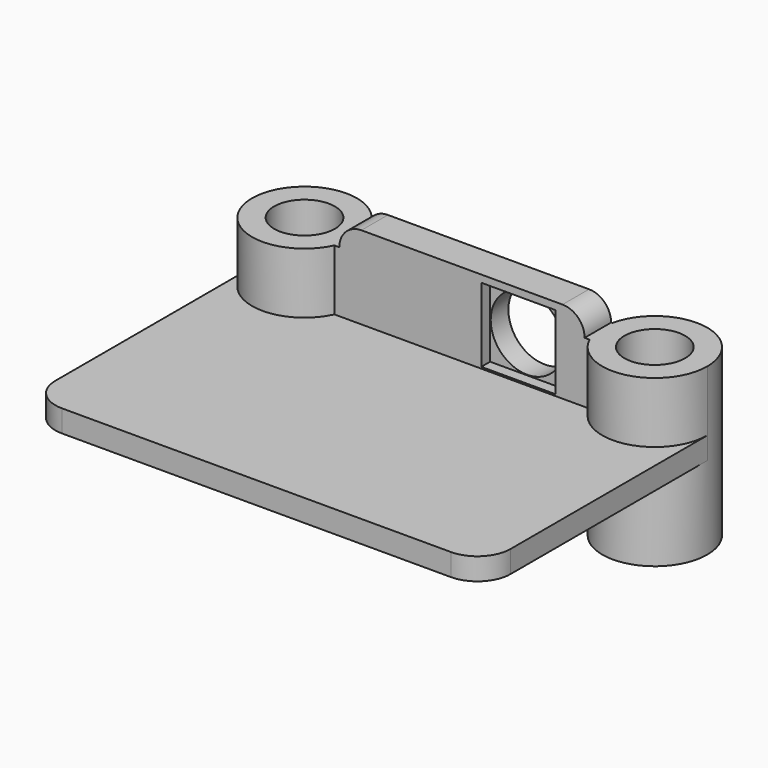
from build123d import *

# Parameters (mm, degrees)
F1_DEPTH      = 2
F0_R          = 2.75
F2_DEPTH      = 7.5
F4_R          = 3.3
F5_DEPTH      = 1
F5_DEPTH_BACK = 2
F7_DEPTH      = 2
F8_W          = 6.7
F8_H          = 6.7
F8_R          = 3.3
F9_DEPTH      = 1


# Not quite as in the source:
# - after a boolean that leaves OpenCascade's solid faulty, fix() repairs it


with BuildPart() as f1:
    # F0 (on Top) → F1 (new body)
    with BuildSketch(Plane.XY):
        with BuildLine():
            ThreePointArc((20.6, 10.25), (12.4912427894, 6.8912427894), (15.85, 15))
            Line((15.85, 15), (-15.85, 15))
            ThreePointArc((-15.85, 15), (-12.4912427894, 13.6087572106), (-11.1, 10.25))
            ThreePointArc((-11.1, 10.25), (-15.85, 5.5), (-20.6, 10.25))
            Line((-20.6, 10.25), (-20.6, -12))
            ThreePointArc((-20.6, -12), (-19.7213203436, -14.1213203436), (-17.6, -15))
            Line((-17.6, -15), (17.6, -15))
            ThreePointArc((17.6, -15), (19.7213203436, -14.1213203436), (20.6, -12))
            Line((20.6, -12), (20.6, 10.25))
        make_face()
    extrude(amount=F1_DEPTH)

    # F0 (on Top) → F2 (join, symmetric)
    with BuildSketch(Plane.XY):
        with BuildLine():
            ThreePointArc((-11.1, 10.25), (-12.4912427894, 13.6087572106), (-15.85, 15))
            ThreePointArc((-15.85, 15), (-19.2087572106, 13.6087572106), (-20.6, 10.25))
            ThreePointArc((-20.6, 10.25), (-15.85, 5.5), (-11.1, 10.25))
        make_face()
        with Locations((-15.85, 10.25)):
            Circle(F0_R, mode=Mode.SUBTRACT)
        with BuildLine():
            ThreePointArc((20.6, 10.25), (19.2087572106, 13.6087572106), (15.85, 15))
            ThreePointArc((15.85, 15), (12.4912427894, 6.8912427894), (20.6, 10.25))
        make_face()
        with Locations((15.85, 10.25)):
            Circle(F0_R, mode=Mode.SUBTRACT)
    extrude(amount=F2_DEPTH, both=True)

    # F4 (on line) → F5 (join, two sides)
    with BuildSketch(Plane(origin=(0, 10.25, 0), x_dir=(-1, 0, 0), z_dir=(0, 1, 0))) as f5_sk:
        with BuildLine():
            Line((-13.1, 7.5), (-13.1, 2))
            Line((-13.1, 2), (-11.1, 2))
            Line((-11.1, 2), (11.1, 2))
            Line((11.1, 2), (13.1, 2))
            Line((13.1, 2), (13.1, 7.5))
            Line((13.1, 7.5), (11.1, 7.5))
            ThreePointArc((11.1, 7.5), (10.5142135624, 8.9142135624), (9.1, 9.5))
            Line((9.1, 9.5), (-9.1, 9.5))
            ThreePointArc((-9.1, 9.5), (-10.5142135624, 8.9142135624), (-11.1, 7.5))
            Line((-11.1, 7.5), (-13.1, 7.5))
        make_face()
        with Locations((-5.1, 5.5)):
            Circle(F4_R, mode=Mode.SUBTRACT)
    extrude(amount=F5_DEPTH)
    extrude(f5_sk.sketch, amount=-F5_DEPTH_BACK)

    # F6 (on face) → F7 (cut, through all)
    with BuildSketch(Plane.XY.offset(2)):
        with BuildLine():
            ThreePointArc((-15.85, 15), (-12.8656659034, 13.9454363748), (-11.2064560947, 11.25))
            Line((-11.2064560947, 11.25), (11.2064560947, 11.25))
            ThreePointArc((11.2064560947, 11.25), (12.8656659034, 13.9454363748), (15.85, 15))
            Line((15.85, 15), (-15.85, 15))
        make_face()
    extrude(amount=-F7_DEPTH, mode=Mode.SUBTRACT)

    # F8 (on face) → F9 (cut)
    with BuildSketch(Plane.XZ.offset(-8.25)):
        with Locations((5.1, 5.5)):
            Rectangle(F8_W, F8_H)
        with Locations((5.1, 5.5)):
            Circle(F8_R, mode=Mode.SUBTRACT)
        with Locations((5.1, 5.5)):
            Circle(F8_R)
    extrude(amount=-F9_DEPTH, mode=Mode.SUBTRACT)

    add(f1.part.fix(), mode=Mode.REPLACE)


solid = f1.part
